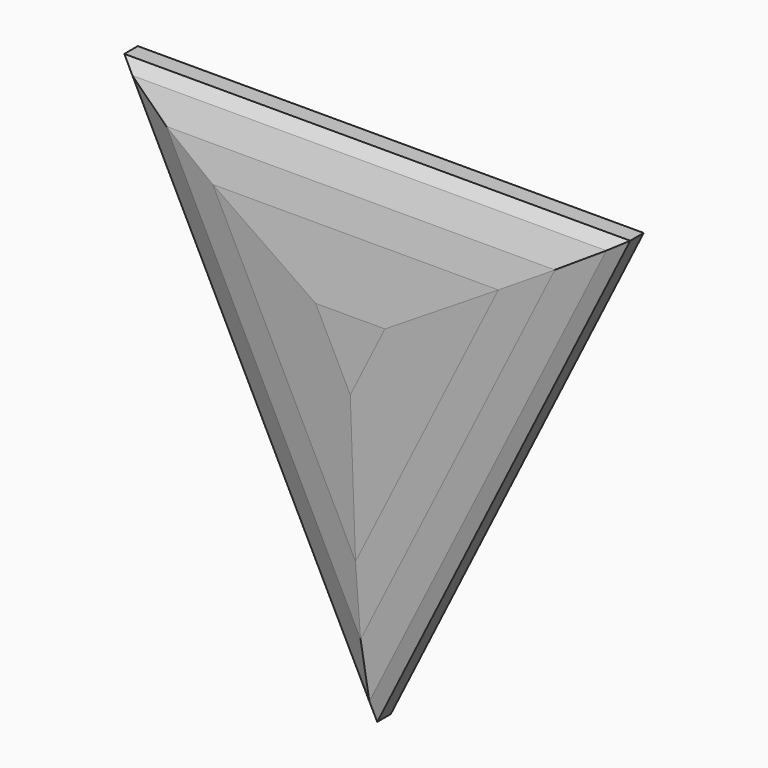
from build123d import *

# Parameters (mm, degrees)
F1_DEPTH = 12.7
F2_SIZE  = 5.08
F3_T     = -2.54
F4_SIZE  = 5.08
F5_SIZE  = 5.08
F6_SIZE  = 5.08


# Not quite as in the source:
# - a feature of the source that left no trace in its solid (it failed there, or was rolled back) is left out


with BuildPart() as f1:
    # F0 (on Front) → F1 (new body)
    with BuildSketch(Plane.XZ):
        Polygon((0, 0), (-38.1, 38.1), (0, -38.1), align=None)
        Polygon((38.1, 38.1), (-38.1, 38.1), (0, 0), align=None)
        Polygon((0, 0), (0, -38.1), (38.1, 38.1), align=None)
    extrude(amount=F1_DEPTH)

    # F2
    f2_edges = [f1.edges().sort_by_distance(p)[0] for p in [
        (0, -12.7, 38.1),
        (-19.05, -12.7, 0),
        (19.05, -12.7, 0),
        (-19.05, 0, 0),
        (0, 0, 38.1),
        (19.05, 0, 0),
    ]]
    chamfer(f2_edges, length=F2_SIZE)

    # F3
    f3_openings = [f1.faces().sort_by_distance(p)[0] for p in [
        (0, 0, 13.099742),
    ]]
    offset(amount=F3_T, openings=f3_openings, kind=Kind.INTERSECTION)

    # F4
    f4_edges = [f1.edges().sort_by_distance(p)[0] for p in [
        (0, -12.7, 33.02),
        (14.940194, -12.7, 3.139613),
        (-14.940194, -12.7, 3.139613),
    ]]
    chamfer(f4_edges, length=F4_SIZE)

    # F5
    f5_edges = [f1.edges().sort_by_distance(p)[0] for p in [
        (0, -12.7, 27.94),
        (10.830387, -12.7, 6.279225),
        (-10.830387, -12.7, 6.279225),
    ]]
    chamfer(f5_edges, length=F5_SIZE)

    # F6
    f6_edges = [f1.edges().sort_by_distance(p)[0] for p in [
        (0, -12.7, 22.86),
        (6.720581, -12.7, 9.418838),
        (-6.720581, -12.7, 9.418838),
    ]]
    chamfer(f6_edges, length=F6_SIZE)


solid = f1.part
